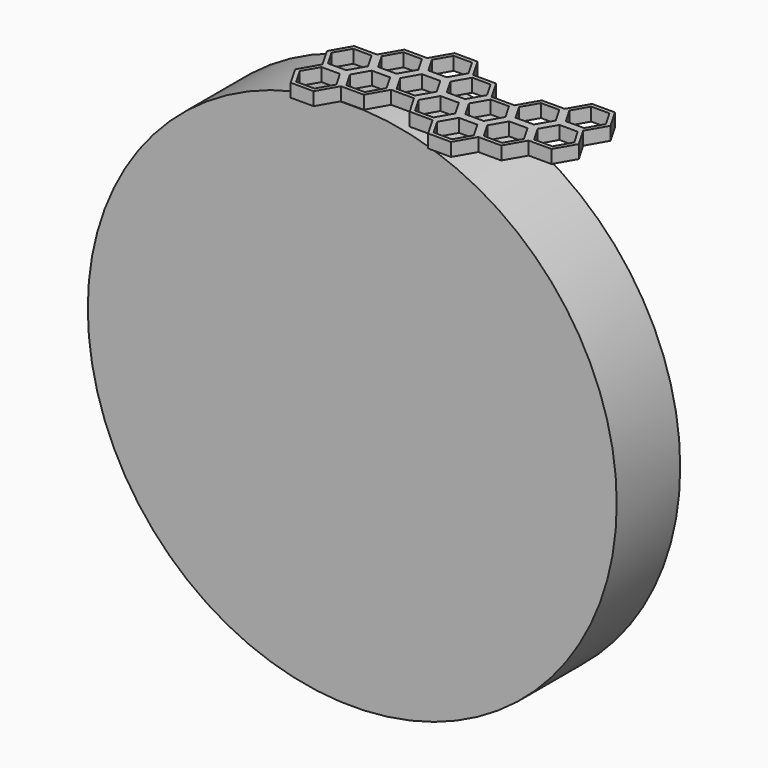
from build123d import *

# Parameters (mm, degrees)
F0_R     = 100
F1_DEPTH = 30
F4_DEPTH = 5


with BuildPart() as f1:
    # F0 (on Front) → F1 (new body)
    with BuildSketch(Plane.XZ):
        Circle(F0_R)
    extrude(amount=F1_DEPTH)


with BuildPart() as f4:
    # F3 (on offset) → F4 (new body)
    with BuildSketch(Plane.XY.offset(100)):
        Polygon((8.6602540378, -22.447098383), (4.3301270189, -14.947098383), (-4.3301270189, -14.947098383), (-8.6602540378, -22.447098383), (-4.3301270189, -29.947098383), (4.3301270189, -29.947098383), align=None)
        Polygon((6.9282032303, -22.447098383), (3.4641016151, -28.447098383), (-3.4641016151, -28.447098383), (-6.9282032303, -22.447098383), (-3.4641016151, -16.447098383), (3.4641016151, -16.447098383), align=None, mode=Mode.SUBTRACT)
        Polygon((-4.3301270189, -14.947098383), (4.3301270189, -14.947098383), (8.6602540378, -7.447098383), (4.3301270189, 0.052901617), (-4.3301270189, 0.052901617), (-8.6602540378, -7.447098383), align=None)
        Polygon((6.9282032303, -7.447098383), (3.4641016151, -13.447098383), (-3.4641016151, -13.447098383), (-6.9282032303, -7.447098383), (-3.4641016151, -1.447098383), (3.4641016151, -1.447098383), align=None, mode=Mode.SUBTRACT)
        Polygon((8.6602540378, -7.447098383), (4.3301270189, -14.947098383), (8.6602540378, -22.447098383), (17.3205080757, -22.447098383), (21.6506350946, -14.947098383), (17.3205080757, -7.447098383), align=None)
        Polygon((19.918584287, -14.947098383), (16.4544826719, -20.947098383), (9.5262794416, -20.947098383), (6.0621778265, -14.947098383), (9.5262794416, -8.947098383), (16.4544826719, -8.947098383), align=None, mode=Mode.SUBTRACT)
        Polygon((-8.6602540378, -22.447098383), (-4.3301270189, -14.947098383), (-8.6602540378, -7.447098383), (-17.3205080757, -7.447098383), (-21.6506350946, -14.947098383), (-17.3205080757, -22.447098383), align=None)
        Polygon((-6.0621778265, -14.947098383), (-9.5262794416, -20.947098383), (-16.4544826719, -20.947098383), (-19.918584287, -14.947098383), (-16.4544826719, -8.947098383), (-9.5262794416, -8.947098383), align=None, mode=Mode.SUBTRACT)
        Polygon((4.3301270189, 0.052901617), (8.6602540378, -7.447098383), (17.3205080757, -7.447098383), (21.6506350946, 0.052901617), (17.3205080757, 7.552901617), (8.6602540378, 7.552901617), align=None)
        Polygon((19.918584287, 0.052901617), (16.4544826719, -5.947098383), (9.5262794416, -5.947098383), (6.0621778265, 0.052901617), (9.5262794416, 6.052901617), (16.4544826719, 6.052901617), align=None, mode=Mode.SUBTRACT)
        Polygon((-4.3301270189, -29.947098383), (-8.6602540378, -22.447098383), (-17.3205080757, -22.447098383), (-21.6506350946, -29.947098383), (-17.3205080757, -37.447098383), (-8.6602540378, -37.447098383), align=None)
        Polygon((-6.0621778265, -29.947098383), (-9.5262794416, -35.947098383), (-16.4544826719, -35.947098383), (-19.918584287, -29.947098383), (-16.4544826719, -23.947098383), (-9.5262794416, -23.947098383), align=None, mode=Mode.SUBTRACT)
        Polygon((21.6506350946, 0.052901617), (17.3205080757, -7.447098383), (21.6506350946, -14.947098383), (30.3108891325, -14.947098383), (34.6410161514, -7.447098383), (30.3108891325, 0.052901617), align=None)
        Polygon((32.9089653438, -7.447098383), (29.4448637287, -13.447098383), (22.5166604984, -13.447098383), (19.0525588833, -7.447098383), (22.5166604984, -1.447098383), (29.4448637287, -1.447098383), align=None, mode=Mode.SUBTRACT)
        Polygon((21.6506350946, -14.947098383), (17.3205080757, -22.447098383), (21.6506350946, -29.947098383), (30.3108891325, -29.947098383), (34.6410161514, -22.447098383), (30.3108891325, -14.947098383), align=None)
        Polygon((32.9089653438, -22.447098383), (29.4448637287, -28.447098383), (22.5166604984, -28.447098383), (19.0525588833, -22.447098383), (22.5166604984, -16.447098383), (29.4448637287, -16.447098383), align=None, mode=Mode.SUBTRACT)
        Polygon((34.6410161514, -7.447098383), (30.3108891325, -14.947098383), (34.6410161514, -22.447098383), (43.3012701892, -22.447098383), (47.6313972081, -14.947098383), (43.3012701892, -7.447098383), align=None)
        Polygon((45.8993464006, -14.947098383), (42.4352447854, -20.947098383), (35.5070415552, -20.947098383), (32.04293994, -14.947098383), (35.5070415552, -8.947098383), (42.4352447854, -8.947098383), align=None, mode=Mode.SUBTRACT)
        Polygon((34.6410161514, -22.447098383), (30.3108891325, -29.947098383), (34.6410161514, -37.447098383), (43.3012701892, -37.447098383), (47.6313972081, -29.947098383), (43.3012701892, -22.447098383), align=None)
        Polygon((45.8993464006, -29.947098383), (42.4352447854, -35.947098383), (35.5070415552, -35.947098383), (32.04293994, -29.947098383), (35.5070415552, -23.947098383), (42.4352447854, -23.947098383), align=None, mode=Mode.SUBTRACT)
        Polygon((47.6313972081, 0.052901617), (43.3012701892, -7.447098383), (47.6313972081, -14.947098383), (56.291651246, -14.947098383), (60.6217782649, -7.447098383), (56.291651246, 0.052901617), align=None)
        Polygon((58.8897274573, -7.447098383), (55.4256258422, -13.447098383), (48.4974226119, -13.447098383), (45.0333209968, -7.447098383), (48.4974226119, -1.447098383), (55.4256258422, -1.447098383), align=None, mode=Mode.SUBTRACT)
        Polygon((47.6313972081, -14.947098383), (43.3012701892, -22.447098383), (47.6313972081, -29.947098383), (56.291651246, -29.947098383), (60.6217782649, -22.447098383), (56.291651246, -14.947098383), align=None)
        Polygon((58.8897274573, -22.447098383), (55.4256258422, -28.447098383), (48.4974226119, -28.447098383), (45.0333209968, -22.447098383), (48.4974226119, -16.447098383), (55.4256258422, -16.447098383), align=None, mode=Mode.SUBTRACT)
        Polygon((60.6217782649, -7.447098383), (56.291651246, -14.947098383), (60.6217782649, -22.447098383), (69.2820323028, -22.447098383), (73.6121593217, -14.947098383), (69.2820323028, -7.447098383), align=None)
        Polygon((71.8801085141, -14.947098383), (68.416006899, -20.947098383), (61.4878036687, -20.947098383), (58.0237020536, -14.947098383), (61.4878036687, -8.947098383), (68.416006899, -8.947098383), align=None, mode=Mode.SUBTRACT)
        Polygon((60.6217782649, 7.552901617), (56.291651246, 0.052901617), (60.6217782649, -7.447098383), (69.2820323028, -7.447098383), (73.6121593217, 0.052901617), (69.2820323028, 7.552901617), align=None)
        Polygon((71.8801085141, 0.052901617), (68.416006899, -5.947098383), (61.4878036687, -5.947098383), (58.0237020536, 0.052901617), (61.4878036687, 6.052901617), (68.416006899, 6.052901617), align=None, mode=Mode.SUBTRACT)
    extrude(amount=F4_DEPTH)


solid = Compound([f1.part, f4.part])
